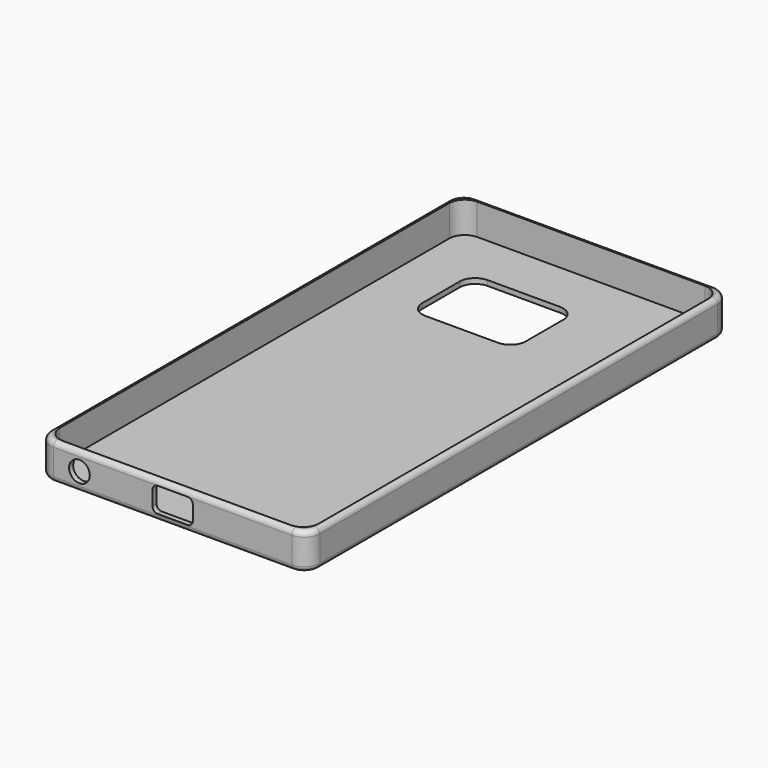
from build123d import *

# Parameters (mm, degrees)
F1_DEPTH = 1
F2_DEPTH = 7
F3_R     = 0.99999
F4_R     = 2
F5_DEPTH = 1


# Not quite as in the source:
# - a fillet or chamfer is up to 0.001 mm smaller than in the source, because OpenCascade refuses the exact size


with BuildPart() as f1:
    # F0 (on Top) → F1 (new body)
    with BuildSketch(Plane.XY):
        with BuildLine():
            Line((26, -48), (26, 48))
            ThreePointArc((26, 48), (25.1213203436, 50.1213203436), (23, 51))
            Line((23, 51), (-23, 51))
            ThreePointArc((-23, 51), (-25.1213203436, 50.1213203436), (-26, 48))
            Line((-26, 48), (-26, -48))
            ThreePointArc((-26, -48), (-25.1213203436, -50.1213203436), (-23, -51))
            Line((-23, -51), (23, -51))
            ThreePointArc((23, -51), (25.1213203436, -50.1213203436), (26, -48))
        make_face()
        with BuildLine():
            ThreePointArc((-25, 47), (-24.1213203436, 49.1213203436), (-22, 50))
            Line((-22, 50), (22, 50))
            ThreePointArc((22, 50), (24.1213203436, 49.1213203436), (25, 47))
            Line((25, 47), (25, -47))
            ThreePointArc((25, -47), (24.1213203436, -49.1213203436), (22, -50))
            Line((22, -50), (-22, -50))
            ThreePointArc((-22, -50), (-24.1213203436, -49.1213203436), (-25, -47))
            Line((-25, -47), (-25, 47))
        make_face(mode=Mode.SUBTRACT)
        with BuildLine():
            Line((22, 50), (-22, 50))
            ThreePointArc((-22, 50), (-24.1213203436, 49.1213203436), (-25, 47))
            Line((-25, 47), (-25, -47))
            ThreePointArc((-25, -47), (-24.1213203436, -49.1213203436), (-22, -50))
            Line((-22, -50), (22, -50))
            ThreePointArc((22, -50), (24.1213203436, -49.1213203436), (25, -47))
            Line((25, -47), (25, 47))
            ThreePointArc((25, 47), (24.1213203436, 49.1213203436), (22, 50))
        make_face()
        with BuildLine():
            ThreePointArc((-15, 37), (-14.1213203436, 39.1213203436), (-12, 40))
            Line((-12, 40), (2, 40))
            ThreePointArc((2, 40), (4.1213203436, 39.1213203436), (5, 37))
            Line((5, 37), (5, 28))
            ThreePointArc((5, 28), (4.1213203436, 25.8786796564), (2, 25))
            Line((2, 25), (-12, 25))
            ThreePointArc((-12, 25), (-14.1213203436, 25.8786796564), (-15, 28))
            Line((-15, 28), (-15, 37))
        make_face(mode=Mode.SUBTRACT)
    extrude(amount=F1_DEPTH)

    # F0 (on Top) → F2 (join)
    with BuildSketch(Plane.XY):
        with BuildLine():
            Line((26, -48), (26, 48))
            ThreePointArc((26, 48), (25.1213203436, 50.1213203436), (23, 51))
            Line((23, 51), (-23, 51))
            ThreePointArc((-23, 51), (-25.1213203436, 50.1213203436), (-26, 48))
            Line((-26, 48), (-26, -48))
            ThreePointArc((-26, -48), (-25.1213203436, -50.1213203436), (-23, -51))
            Line((-23, -51), (23, -51))
            ThreePointArc((23, -51), (25.1213203436, -50.1213203436), (26, -48))
        make_face()
        with BuildLine():
            ThreePointArc((-25, 47), (-24.1213203436, 49.1213203436), (-22, 50))
            Line((-22, 50), (22, 50))
            ThreePointArc((22, 50), (24.1213203436, 49.1213203436), (25, 47))
            Line((25, 47), (25, -47))
            ThreePointArc((25, -47), (24.1213203436, -49.1213203436), (22, -50))
            Line((22, -50), (-22, -50))
            ThreePointArc((-22, -50), (-24.1213203436, -49.1213203436), (-25, -47))
            Line((-25, -47), (-25, 47))
        make_face(mode=Mode.SUBTRACT)
    extrude(amount=F2_DEPTH)

    # F3 (radius 1 in the source; OpenCascade refuses exactly that, so slightly less here)
    f3_edges = [f1.edges().sort_by_distance(p)[0] for p in [
        (26, 0, 0),
        (-26, 0, 7),
    ]]
    fillet(f3_edges, radius=F3_R)

    # F4 (on face) → F5 (cut, through all)
    with BuildSketch(Plane.XZ.offset(51)):
        with BuildLine():
            Line((2.9, 6), (-2.9, 6))
            ThreePointArc((-2.9, 6), (-3.6071067812, 5.7071067812), (-3.9, 5))
            Line((-3.9, 5), (-3.9, 2.2120511904))
            ThreePointArc((-3.9, 2.2120511904), (-3.6071067812, 1.5049444092), (-2.9, 1.2120511904))
            Line((-2.9, 1.2120511904), (2.9, 1.2120511904))
            ThreePointArc((2.9, 1.2120511904), (3.6071067812, 1.5049444092), (3.9, 2.2120511904))
            Line((3.9, 2.2120511904), (3.9, 5))
            ThreePointArc((3.9, 5), (3.6071067812, 5.7071067812), (2.9, 6))
        make_face()
        with Locations((-18, 3.5)):
            Circle(F4_R)
    extrude(amount=-F5_DEPTH, mode=Mode.SUBTRACT)


solid = f1.part
